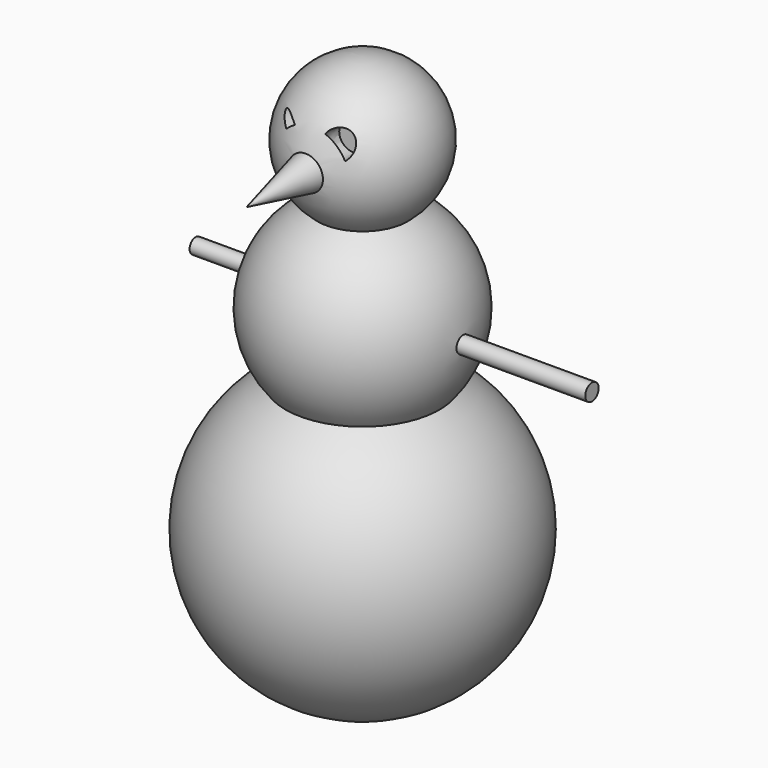
from build123d import *

# Parameters (mm, degrees)
F6_DEPTH = 3.302
F7_W     = 13.8215459883
F7_H     = 1.2585521908
F7_W_2   = 37.9781834781
F7_H_2   = 1.381920767


with BuildPart() as f1:
    # F0 (on Front) → F1 (revolve)
    with BuildSketch(Plane.XZ):
        with BuildLine():
            ThreePointArc((0, 36.5393093155), (-11.4251104851, 28.3988603898), (-7.4618768804, 14.9417864989))
            ThreePointArc((-7.4618768804, 14.9417864989), (-16.356873737, 3.3747995359), (-12.7664426916, -10.7682185787))
            ThreePointArc((-12.7664426916, -10.7682185787), (-24.1091703633, -38.8838765875), (0, -57.2658133922))
            Line((0, -57.2658133922), (0, 36.5393093155))
        make_face()
    revolve(axis=Axis((0, 0, -10.3632520383), (0, 0, -1)))

    # F2 (on Right) → F3 (revolve)
    with BuildSketch(Plane.YZ):
        Polygon((-24.0200255066, 24.3646577001), (-11.4886462688, 24.3646577001), (-11.3669829443, 27.2845905274), align=None)
    revolve(axis=Axis((0, -17.7543358877, 24.3646577001), (0, -1, 0)))

    # F5 (on offset) → F6 (cut)
    with BuildSketch(Plane.XZ.offset(10.414)):
        with BuildLine():
            add(Edge.make_bspline(
                [(-5.6940768845, 30.6755248457), (-6.4590711966, 29.4584885127), (-2.8828964047, 28.0595520455), (0.6932783872, 26.6606155783), (-2.1179020926, 29.2765883785), (-4.9290825725, 31.8925611787), (-5.6940768845, 30.6755248457)],
                knots=[0, 0, 0, 2.0943951024, 2.0943951024, 4.1887902048, 4.1887902048, 6.2831853072, 6.2831853072, 6.2831853072], degree=2, weights=[1, 0.5, 1, 0.5, 1, 0.5, 1]))
        make_face()
        with BuildLine():
            add(Edge.make_bspline(
                [(5.3165038116, 30.7971872389), (2.1750298927, 33.0720474057), (1.8295611088, 29.2884281393), (1.484092325, 25.5048088729), (4.9710350278, 27.0135679726), (8.4579777306, 28.5223270722), (5.3165038116, 30.7971872389)],
                knots=[4.7123889804, 4.7123889804, 4.7123889804, 6.8067840828, 6.8067840828, 8.9011791852, 8.9011791852, 10.9955742876, 10.9955742876, 10.9955742876], degree=2, weights=[1, 0.5, 1, 0.5, 1, 0.5, 1]))
        make_face()
    extrude(amount=-F6_DEPTH, mode=Mode.SUBTRACT)

    # F7 (on Front) → F8 (revolve)
    with BuildSketch(Plane.XZ):
        with Locations((-20.7323189825, 0.6292760954)):
            Rectangle(F7_W, F7_H)
        with Locations((18.9890917391, 0.6909603835)):
            Rectangle(F7_W_2, F7_H_2)
    revolve(axis=Axis((-13.8215459883, 0, 0), (-1, 0, 0)))


solid = f1.part
